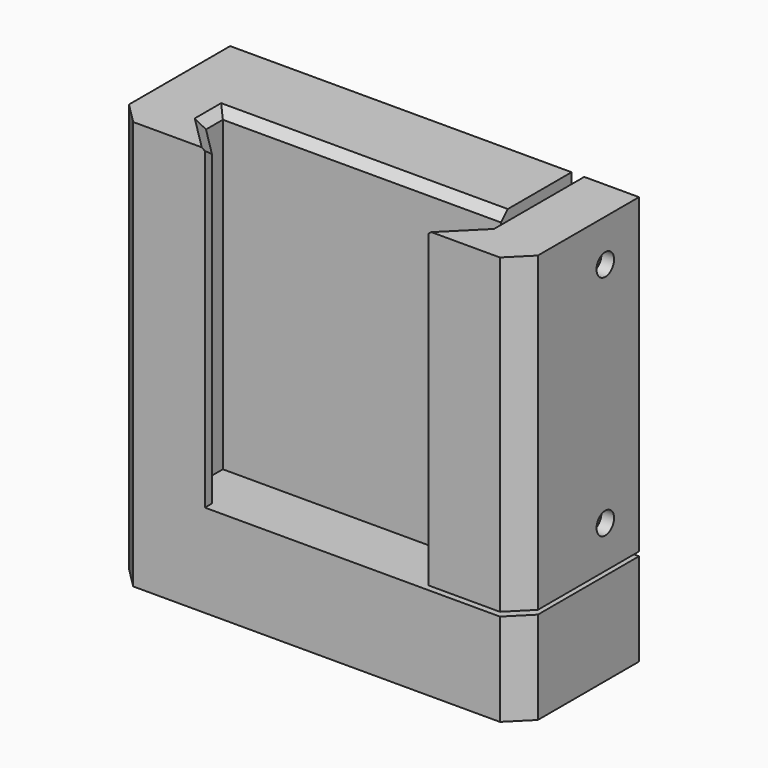
from build123d import *

# Parameters (mm, degrees)
F1_DEPTH      = 37.5
F2_DEPTH      = 37.5
F2_DEPTH_BACK = 36.5
F3_W          = 97
F3_H          = 35
F4_DEPTH      = 22
F5_SIZE       = 5
F5_2_SIZE     = 5
F7_START      = -3
F6_R          = 5.1
F7_DEPTH      = 12
F8_R          = 2.6
F9_DEPTH      = 3
F10_R         = 5.1
F11_DEPTH     = 40
F12_R         = 5
F13_DEPTH     = 50
F14_SIZE      = 2
F14_2_SIZE    = 2


# Not quite as in the source:
# - a feature names something its author has since deleted; it is built from what else it names


with BuildPart() as f1:
    # F0 (on Top) → F1 (new body, symmetric)
    with BuildSketch(Plane.XY):
        Polygon((-26.5, -15), (-26.5, -12.9124395503), (-33.5, -5.9124395503), (-33.5, -0.9124395503), (32.5, -0.9124395503), (32.5, 20), (-48.5, 20), (-48.5, -15), align=None)
    extrude(amount=F1_DEPTH, both=True)

    # F3 (on face) → F4 (join)
    with BuildSketch(Plane(origin=(0, 0, -37.5), x_dir=(1, 0, 0), z_dir=(0, 0, -1))):
        with Locations((0, -2.5)):
            Rectangle(F3_W, F3_H)
    extrude(amount=F4_DEPTH)

    # F5
    f5_edges = [f1.edges().sort_by_distance(p)[0] for p in [
        (-48.5, -15, -11),
        (48.5, -15, -48.5),
    ]]
    chamfer(f5_edges, length=F5_SIZE)

    # F10 (on face) → F11 (cut)
    with BuildSketch(Plane.YZ.offset(32.5)):
        with Locations((10, 27.5)):
            Circle(F10_R)
        with Locations((10, -26.5)):
            Circle(F10_R)
    extrude(amount=-F11_DEPTH, mode=Mode.SUBTRACT)

    # F14
    f14_edges = [f1.edges().sort_by_distance(p)[0] for p in [
        (-0.5, -0.91244, 37.5),
        (-33.5, -3.41244, 37.5),
        (-30, -9.41244, 37.5),
    ]]
    chamfer(f14_edges, length=F14_SIZE)


with BuildPart() as f2:
    # F0 (on Top) → F2 (new body, two sides)
    with BuildSketch(Plane.XY) as f2_sk:
        Polygon((26.5, -12.9124395503), (26.5, -15), (48.5, -15), (48.5, 20), (33.5, 20), (33.5, -5.9124395503), align=None)
    extrude(amount=F2_DEPTH)
    extrude(f2_sk.sketch, amount=-F2_DEPTH_BACK)

    # F5#2
    f5_2_edges = [f2.edges().sort_by_distance(p)[0] for p in [
        (48.5, -15, 0.5),
    ]]
    chamfer(f5_2_edges, length=F5_2_SIZE)

    # F6 (on face) → F7 (cut)
    with BuildSketch(Plane.YZ.offset(48.5).offset(F7_START)):
        with Locations((10, 27.5)):
            Circle(F6_R)
        with Locations((10, -26.5)):
            Circle(F6_R)
    extrude(amount=-F7_DEPTH, mode=Mode.SUBTRACT)

    # F8 (on face) → F9 (cut)
    with BuildSketch(Plane.YZ.offset(48.5)):
        with Locations((10, 27.5)):
            Circle(F8_R)
        with Locations((10, -26.5)):
            Circle(F8_R)
    extrude(amount=-F9_DEPTH, mode=Mode.SUBTRACT)

    # F14#2
    f14_2_edges = [f2.edges().sort_by_distance(p)[0] for p in [
        (30, -9.41244, 37.5),
        (33.5, 7.04378, 37.5),
    ]]
    chamfer(f14_2_edges, length=F14_2_SIZE)


with BuildPart() as f13:
    # F12 (on face) → F13 (new body)
    with BuildSketch(Plane(origin=(45.5, 0, 0), x_dir=(0, -1, 0), z_dir=(-1, 0, 0))):
        with Locations((-10, 27.5)):
            Circle(F12_R)
    extrude(amount=F13_DEPTH)


with BuildPart() as f13b:
    # F12 (on face) → F13, piece 2 (new body)
    with BuildSketch(Plane(origin=(45.5, 0, 0), x_dir=(0, -1, 0), z_dir=(-1, 0, 0))):
        with Locations((-10, -26.5)):
            Circle(F12_R)
    extrude(amount=F13_DEPTH)


solid = Compound([f1.part, f2.part, f13.part, f13b.part])
